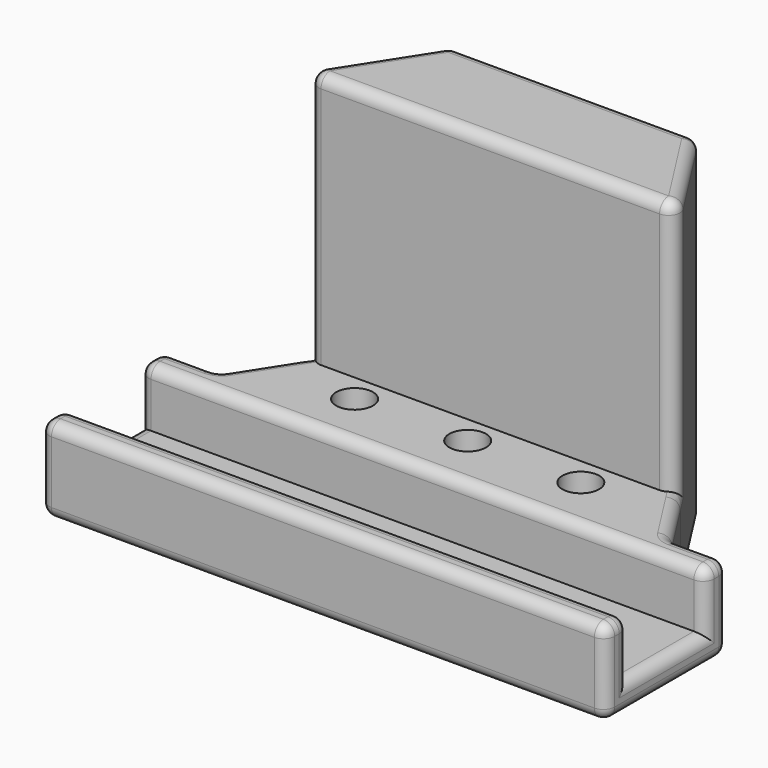
from build123d import *

# Parameters (mm, degrees)
F0_R     = 3.25
F0_W     = 100
F0_H     = 17
F0_H_2   = 5
F1_DEPTH = 5
F2_DEPTH = 15
F3_DEPTH = 60
F4_START = 55
F4_DEPTH = 5
F5_R     = 2


with BuildPart() as f1:
    # F0 (on Top) → F1 (new body)
    with BuildSketch(Plane.XY):
        Polygon((-21.7332131192, 42), (-33.5906010945, 23.5), (33.5906010945, 23.5), (21.7332131192, 42), align=None)
        with BuildLine():
            ThreePointArc((-20.5, 35), (-19.9142135624, 36.4142135624), (-18.5, 37))
            Line((-18.5, 37), (18.5, 37))
            ThreePointArc((18.5, 37), (19.9142135624, 36.4142135624), (20.5, 35))
            Line((20.5, 35), (20.5, 30.5))
            ThreePointArc((20.5, 30.5), (19.9142135624, 29.0857864376), (18.5, 28.5))
            Line((18.5, 28.5), (-18.5, 28.5))
            ThreePointArc((-18.5, 28.5), (-19.9142135624, 29.0857864376), (-20.5, 30.5))
            Line((-20.5, 30.5), (-20.5, 35))
        make_face(mode=Mode.SUBTRACT)
        Polygon((-33.5906010945, 23.5), (-40, 13.5), (40, 13.5), (33.5906010945, 23.5), align=None)
        with Locations((-20, 18.5)):
            Circle(F0_R, mode=Mode.SUBTRACT)
        with Locations((0, 18.5)):
            Circle(F0_R, mode=Mode.SUBTRACT)
        with Locations((20, 18.5)):
            Circle(F0_R, mode=Mode.SUBTRACT)
        with Locations((-20, 18.5)):
            Circle(F0_R)
        with Locations((0, 18.5)):
            Circle(F0_R)
        with Locations((20, 18.5)):
            Circle(F0_R)
        Polygon((-40, 13.5), (-50, 13.5), (-50, 8.5), (50, 8.5), (50, 13.5), (40, 13.5), align=None)
        Rectangle(F0_W, F0_H)
        with Locations((0, -11)):
            Rectangle(F0_W, F0_H_2)
    extrude(amount=F1_DEPTH)

    # F0 (on Top) → F2 (join)
    with BuildSketch(Plane.XY):
        Polygon((-33.5906010945, 23.5), (-40, 13.5), (40, 13.5), (33.5906010945, 23.5), align=None)
        with Locations((-20, 18.5)):
            Circle(F0_R, mode=Mode.SUBTRACT)
        with Locations((0, 18.5)):
            Circle(F0_R, mode=Mode.SUBTRACT)
        with Locations((20, 18.5)):
            Circle(F0_R, mode=Mode.SUBTRACT)
        Polygon((-40, 13.5), (-50, 13.5), (-50, 8.5), (50, 8.5), (50, 13.5), (40, 13.5), align=None)
        with Locations((0, -11)):
            Rectangle(F0_W, F0_H_2)
    extrude(amount=F2_DEPTH)

    # F0 (on Top) → F3 (join)
    with BuildSketch(Plane.XY):
        Polygon((-21.7332131192, 42), (-33.5906010945, 23.5), (33.5906010945, 23.5), (21.7332131192, 42), align=None)
        with BuildLine():
            ThreePointArc((-20.5, 35), (-19.9142135624, 36.4142135624), (-18.5, 37))
            Line((-18.5, 37), (18.5, 37))
            ThreePointArc((18.5, 37), (19.9142135624, 36.4142135624), (20.5, 35))
            Line((20.5, 35), (20.5, 30.5))
            ThreePointArc((20.5, 30.5), (19.9142135624, 29.0857864376), (18.5, 28.5))
            Line((18.5, 28.5), (-18.5, 28.5))
            ThreePointArc((-18.5, 28.5), (-19.9142135624, 29.0857864376), (-20.5, 30.5))
            Line((-20.5, 30.5), (-20.5, 35))
        make_face(mode=Mode.SUBTRACT)
    extrude(amount=F3_DEPTH)

    # F0 (on Top) → F4 (join)
    with BuildSketch(Plane.XY.offset(F4_START)):
        with BuildLine():
            Line((18.5, 37), (-18.5, 37))
            ThreePointArc((-18.5, 37), (-19.9142135624, 36.4142135624), (-20.5, 35))
            Line((-20.5, 35), (-20.5, 30.5))
            ThreePointArc((-20.5, 30.5), (-19.9142135624, 29.0857864376), (-18.5, 28.5))
            Line((-18.5, 28.5), (18.5, 28.5))
            ThreePointArc((18.5, 28.5), (19.9142135624, 29.0857864376), (20.5, 30.5))
            Line((20.5, 30.5), (20.5, 35))
            ThreePointArc((20.5, 35), (19.9142135624, 36.4142135624), (18.5, 37))
        make_face()
    extrude(amount=F4_DEPTH)

    # F5
    f5_edges = [f1.edges().sort_by_distance(p)[0] for p in [
        (0, 42, 0),
        (-30.866607, 27.75, 0),
        (-45, 13.5, 0),
        (-50, 0, 0),
        (0, -13.5, 0),
        (50, 0, 0),
        (45, 13.5, 0),
        (30.866607, 27.75, 0),
        (-19.914214, 36.414214, 0),
        (0, 37, 0),
        (19.914214, 36.414214, 0),
        (20.5, 32.75, 0),
        (19.914214, 29.085786, 0),
        (0, 28.5, 0),
        (-19.914214, 29.085786, 0),
        (-20.5, 32.75, 0),
        (-21.733213, 42, 30),
        (-27.661907, 32.75, 60),
        (-33.590601, 23.5, 37.5),
        (-36.795301, 18.5, 15),
        (-40, 13.5, 7.5),
        (-50, 13.5, 7.5),
        (-50, 11, 15),
        (-50, 8.5, 10),
        (-50, 0, 5),
        (-50, -8.5, 10),
        (-50, -11, 15),
        (-50, -13.5, 7.5),
        (40, 13.5, 7.5),
        (36.795301, 18.5, 15),
        (33.590601, 23.5, 37.5),
        (27.661907, 32.75, 60),
        (21.733213, 42, 30),
        (50, -13.5, 7.5),
        (50, -11, 15),
        (50, -8.5, 10),
        (50, 0, 5),
        (50, 8.5, 10),
        (50, 11, 15),
        (50, 13.5, 7.5),
        (0, 42, 60),
        (0, 23.5, 60),
        (0, -8.5, 15),
        (0, -13.5, 15),
        (0, 8.5, 15),
        (45, 13.5, 15),
        (-45, 13.5, 15),
    ]]
    fillet(f5_edges, radius=F5_R)


solid = f1.part
